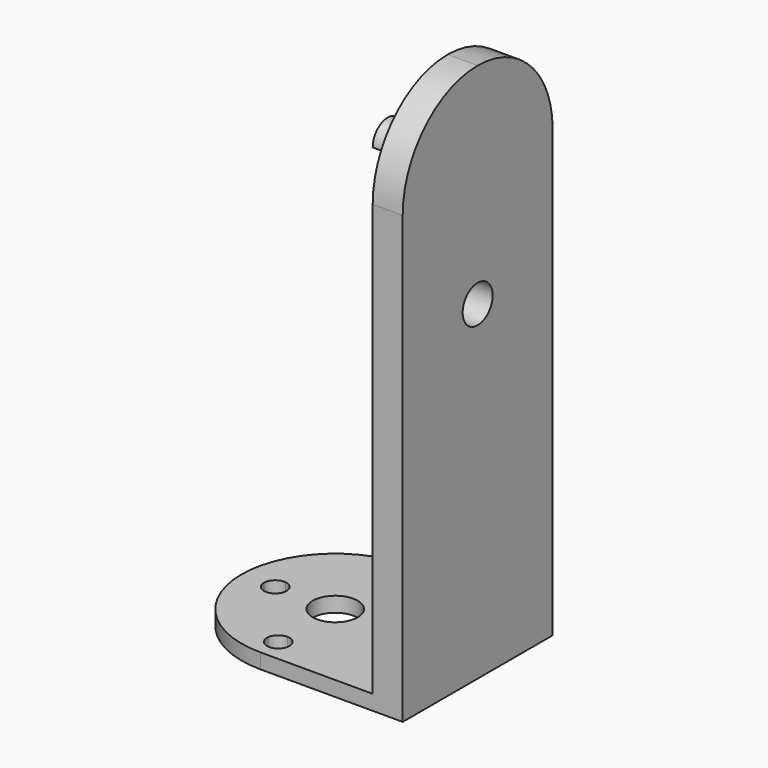
from build123d import *

# Parameters (mm, degrees)
F0_R     = 3
F1_DEPTH = 2
F2_W     = 4
F2_H     = 25
F3_DEPTH = 70
F5_DEPTH = 8
F6_R     = 12.49999
F7_R     = 2.5
F8_DEPTH = 4


# Not quite as in the source:
# - a fillet or chamfer is up to 0.001 mm smaller than in the source, because OpenCascade refuses the exact size
# - a feature names something its author has since deleted; it is built from what else it names


with BuildPart() as f1:
    # F0 (on Top) → F1 (new body)
    with BuildSketch(Plane.XY):
        with BuildLine():
            ThreePointArc((0, -12.5), (8.8388347648, -8.8388347648), (12.5, 0))
            ThreePointArc((12.5, 0), (8.8388347648, 8.8388347648), (0, 12.5))
            ThreePointArc((0, 12.5), (-12.5, 0), (0, -12.5))
        make_face()
        with BuildLine():
            ThreePointArc((1.4953181783, 9.3815789474), (7.2268777039, 6.1662175321), (9.5, 0))
            ThreePointArc((9.5, 0), (7.2268777039, -6.1662175321), (1.4953181783, -9.3815789474))
            ThreePointArc((1.4953181783, -9.3815789474), (1.4988290876, -9.4407432173), (1.5, -9.5))
            ThreePointArc((1.5, -9.5), (-0.0592567827, -10.9988290876), (-1.4953181783, -9.3815789474))
            ThreePointArc((-1.4953181783, -9.3815789474), (-7.2268777039, -6.1662175321), (-9.5, 0))
            ThreePointArc((-9.5, 0), (-7.2268777039, 6.1662175321), (-1.4953181783, 9.3815789474))
            ThreePointArc((-1.4953181783, 9.3815789474), (-0.0592567827, 10.9988290876), (1.5, 9.5))
            ThreePointArc((1.5, 9.5), (1.4988290876, 9.4407432173), (1.4953181783, 9.3815789474))
        make_face(mode=Mode.SUBTRACT)
        with BuildLine():
            ThreePointArc((0, 12.5), (8.8388347648, 8.8388347648), (12.5, 0))
            ThreePointArc((12.5, 0), (8.8388347648, -8.8388347648), (0, -12.5))
            Line((0, -12.5), (19, -12.5))
            Line((19, -12.5), (19, 12.5))
            Line((19, 12.5), (0, 12.5))
        make_face()
        with BuildLine():
            ThreePointArc((7.859375, -1.4933936552), (6.5, 0), (7.859375, 1.4933936552))
            ThreePointArc((7.859375, 1.4933936552), (5.1016100823, 6.1622702446), (1.34e-08, 8))
            ThreePointArc((1.34e-08, 8), (-5.101610072, 6.1622702532), (-7.859375, 1.4933936552))
            ThreePointArc((-7.859375, 1.4933936552), (-6.8907350407, 1.0097184013), (-6.5, 0))
            ThreePointArc((-6.5, 0), (-6.8907350407, -1.0097184013), (-7.859375, -1.4933936552))
            ThreePointArc((-7.859375, -1.4933936552), (-5.1016100771, -6.1622702489), (0, -8))
            ThreePointArc((0, -8), (5.1016100771, -6.1622702489), (7.859375, -1.4933936552))
        make_face()
        Circle(F0_R, mode=Mode.SUBTRACT)
        with BuildLine():
            ThreePointArc((7.859375, 1.4933936552), (9.0097184013, 1.1092649593), (9.5, 0))
            ThreePointArc((9.5, 0), (7.2268777039, 6.1662175321), (1.4953181783, 9.3815789474))
            ThreePointArc((1.4953181783, 9.3815789474), (1.0179313437, 8.3982669201), (1.34e-08, 8))
            ThreePointArc((1.34e-08, 8), (5.1016100823, 6.1622702446), (7.859375, 1.4933936552))
        make_face()
        with BuildLine():
            ThreePointArc((1.4953181783, -9.3815789474), (7.2268777039, -6.1662175321), (9.5, 0))
            ThreePointArc((9.5, 0), (9.0097184013, -1.1092649593), (7.859375, -1.4933936552))
            ThreePointArc((7.859375, -1.4933936552), (5.1016100771, -6.1622702489), (0, -8))
            ThreePointArc((0, -8), (1.0179313388, -8.3982669155), (1.4953181783, -9.3815789474))
        make_face()
        with BuildLine():
            ThreePointArc((1.34e-08, 8), (-1.0179313339, 8.3982669109), (-1.4953181783, 9.3815789474))
            ThreePointArc((-1.4953181783, 9.3815789474), (-7.2268777039, 6.1662175321), (-9.5, 0))
            ThreePointArc((-9.5, 0), (-9.0097184013, 1.1092649593), (-7.859375, 1.4933936552))
            ThreePointArc((-7.859375, 1.4933936552), (-5.101610072, 6.1622702532), (1.34e-08, 8))
        make_face()
        with BuildLine():
            ThreePointArc((-9.5, 0), (-7.2268777039, -6.1662175321), (-1.4953181783, -9.3815789474))
            ThreePointArc((-1.4953181783, -9.3815789474), (-1.0179313388, -8.3982669155), (0, -8))
            ThreePointArc((0, -8), (-5.1016100771, -6.1622702489), (-7.859375, -1.4933936552))
            ThreePointArc((-7.859375, -1.4933936552), (-9.0097184013, -1.1092649593), (-9.5, 0))
        make_face()
    extrude(amount=F1_DEPTH)

    # F2 (on face) → F3 (join)
    with BuildSketch(Plane.XY.offset(2)):
        with Locations((17, 0)):
            Rectangle(F2_W, F2_H)
    extrude(amount=F3_DEPTH)

    # F4 (on face) → F5 (join)
    with BuildSketch(Plane(origin=(15, 0, 0), x_dir=(0, -1, 0), z_dir=(-1, 0, 0))):
        with BuildLine():
            Line((-2.5, 59.5), (2.5, 59.5))
            ThreePointArc((2.5, 59.5), (0, 62), (-2.5, 59.5))
        make_face()
    extrude(amount=F5_DEPTH)

    # F6 (radius 12.5 in the source; OpenCascade refuses exactly that, so slightly less here)
    f6_edges = [f1.edges().sort_by_distance(p)[0] for p in [
        (17, -12.5, 72),
        (17, 12.5, 72),
    ]]
    fillet(f6_edges, radius=F6_R)

    # F7 (on face) → F8 (cut, through all)
    with BuildSketch(Plane.YZ.offset(19)):
        with Locations((0, 44)):
            Circle(F7_R)
    extrude(amount=-F8_DEPTH, mode=Mode.SUBTRACT)


solid = f1.part
